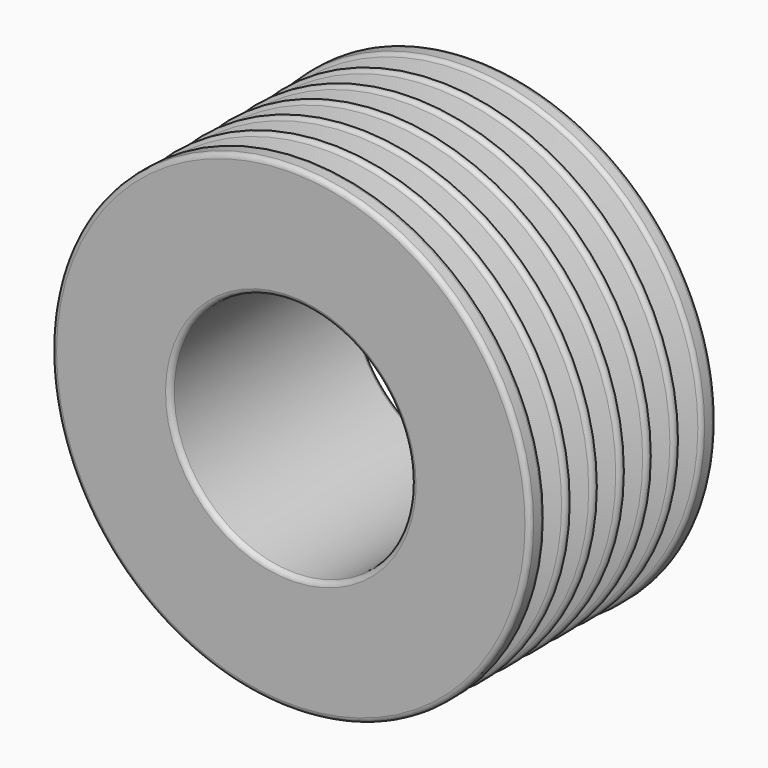
from build123d import *

# Parameters (mm, degrees)
F3_R = 0.508


with BuildPart() as f2:
    # F2: sweep along a path in F0
    with BuildLine(Plane.XZ) as f2_path:
        CenterArc((0, 0), 25.4, 0, 360)
    # F1 (on Right) → F2 (sweep)
    with BuildSketch(Plane.YZ):
        with BuildLine():
            Line((-24.3618413806, 12.7168288454), (0.0262497924, 12.7168288454))
            Line((0.0262497924, 12.7168288454), (0.0262497924, 25.390578095))
            Line((0.0262497924, 25.390578095), (-1.4897372673, 25.390578095))
            ThreePointArc((-1.4897372673, 25.390578095), (-1.782985913, 25.299625112), (-1.970273827, 25.0563342354))
            Line((-1.970273827, 25.0563342354), (-3.0449343395, 22.1037287434))
            ThreePointArc((-3.0449343395, 22.1037287434), (-3.2630920057, 21.9374324407), (-3.505187821, 22.0664163306))
            ThreePointArc((-3.505187821, 22.0664163306), (-3.5144515996, 22.084625219), (-3.5222220071, 22.1035197151))
            Line((-3.5222220071, 22.1035197151), (-4.5544351117, 24.9317915062))
            ThreePointArc((-4.5544351117, 24.9317915062), (-5.0320915531, 25.2656270218), (-5.5091624481, 24.9309552594))
            Line((-5.5091624481, 24.9309552594), (-6.5750335074, 21.9944983557))
            ThreePointArc((-6.5750335074, 21.9944983557), (-6.813568955, 21.8271624745), (-7.0523971757, 21.9940802323))
            Line((-7.0523971757, 21.9940802323), (-8.1181520949, 24.9142568519))
            ThreePointArc((-8.1181520949, 24.9142568519), (-8.5955860575, 25.2480925136), (-9.0727274301, 24.9138387952))
            Line((-9.0727274301, 24.9138387952), (-10.1336001047, 21.9991150768))
            ThreePointArc((-10.1336001047, 21.9991150768), (-10.3722820303, 21.8319881932), (-10.610963956, 21.9991150768))
            Line((-10.610963956, 21.9991150768), (-11.6716756767, 24.9133965778))
            ThreePointArc((-11.6716756767, 24.9133965778), (-12.1490395281, 25.247650345), (-12.6264033794, 24.9133965778))
            Line((-12.6264033794, 24.9133965778), (-13.6896001047, 21.9922875828))
            ThreePointArc((-13.6896001047, 21.9922875828), (-13.9282820303, 21.8251606992), (-14.166963956, 21.9922875828))
            Line((-14.166963956, 21.9922875828), (-15.2276756767, 24.9065690839))
            ThreePointArc((-15.2276756767, 24.9065690839), (-15.7050395281, 25.2408228511), (-16.1824033794, 24.9065690839))
            Line((-16.1824033794, 24.9065690839), (-17.2508460749, 21.971046904))
            ThreePointArc((-17.2508460749, 21.971046904), (-17.4895280006, 21.8039200204), (-17.7282099263, 21.971046904))
            Line((-17.7282099263, 21.971046904), (-18.7914066515, 24.892155899))
            ThreePointArc((-18.7914066515, 24.892155899), (-19.2685480241, 25.2264096175), (-19.7459819867, 24.8925739558))
            Line((-19.7459819867, 24.8925739558), (-20.8094072633, 21.9787805747))
            ThreePointArc((-20.8094072633, 21.9787805747), (-21.0481242446, 21.8118627439), (-21.2866949309, 21.9789896031))
            Line((-21.2866949309, 21.9789896031), (-22.3474066515, 24.8932711042))
            ThreePointArc((-22.3474066515, 24.8932711042), (-22.5333936732, 25.1356541099), (-22.8247705029, 25.2275248714))
            Line((-22.8247705029, 25.2275248714), (-24.3618413806, 25.2275248714))
            Line((-24.3618413806, 25.2275248714), (-24.3618413806, 21.9817499781))
            Line((-24.3618413806, 21.9817499781), (-24.3618413806, 12.7168288454))
        make_face()
    sweep(path=f2_path.line)

    # F3
    f3_edges = [f2.edges().sort_by_distance(p)[0] for p in [
        (-25.390578, 0.02625, 0),
        (25.390578, -0.731744, 0),
        (-25.390578, -1.489737, 0),
        (-25.227525, -22.824771, 0),
        (25.227525, -23.593306, 0),
        (-25.227525, -24.361841, 0),
        (-12.716829, 0.02625, 0),
        (-12.716829, -24.361841, 0),
    ]]
    fillet(f3_edges, radius=F3_R)


solid = f2.part
